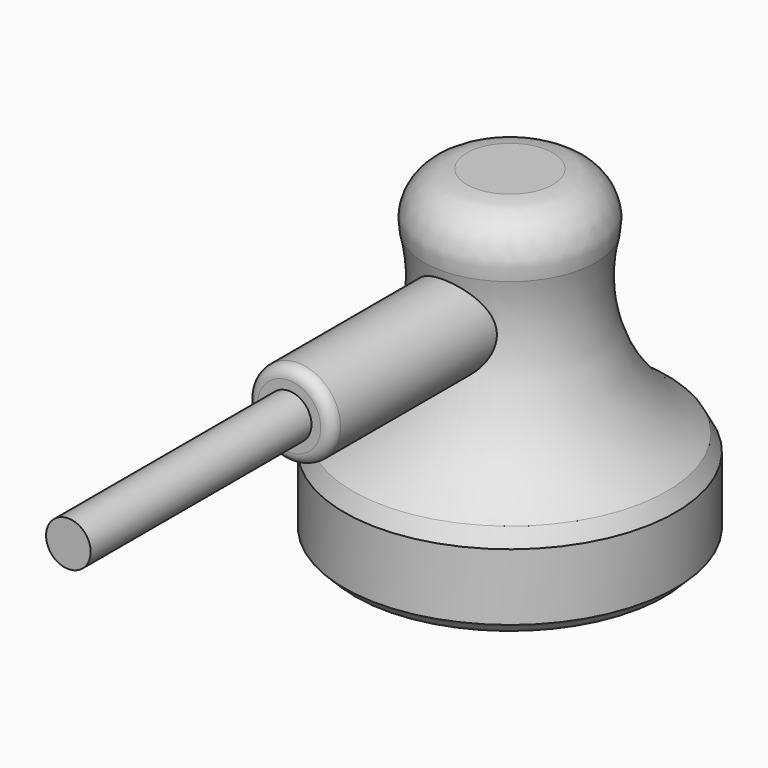
from build123d import *

# Parameters (mm, degrees)
F2_R     = 3.8609958539
F3_DEPTH = 25
F4_R     = 2.0215779579
F5_DEPTH = 25
F6_R     = 4
F8_R     = 1
F9_SIZE  = 1


# Not quite as in the source:
# - a fillet or chamfer that OpenCascade refuses, or shapes differently, is made with other operations: its cross-section is extruded or revolved along the edge and cut away or added


with BuildPart() as f1:
    # F0 (on Front) → F1 (revolve)
    with BuildSketch(Plane.XZ):
        with BuildLine():
            Line((0, 9.6684011082), (0, 39.240504275))
            Line((0, 39.240504275), (-10, 39.240504275))
            ThreePointArc((-10, 39.240504275), (-7.7458675852, 27.3525359295), (-15, 17.6684011082))
            Line((-15, 17.6684011082), (-15, 9.6684011082))
            Line((-15, 9.6684011082), (0, 9.6684011082))
        make_face()
    revolve(axis=Axis((0, 0, 24.4544526916), (0, 0, 1)))

    # F2 (on Front) → F3 (join)
    with BuildSketch(Plane.XZ):
        with Locations((0, 29.6669229865)):
            Circle(F2_R)
    extrude(amount=F3_DEPTH)

    # F4 (on face) → F5 (join)
    with BuildSketch(Plane.XZ.offset(25)):
        with Locations((0, 29.6669229865)):
            Circle(F4_R)
    extrude(amount=F5_DEPTH)

    # F6
    f6_edges = [f1.edges().sort_by_distance(p)[0] for p in [
        (10, 0, 39.240504),
    ]]
    fillet(f6_edges, radius=F6_R)

    # F7: chamfer of 1 on 1 edges, made by hand

    # F7_s1 → F7_t2 (revolve, cut)
    with BuildSketch(Plane.XZ):
        with BuildLine():
            Line((-14.1986684737, 18.1758192127), (-15.0191266727, 16.668849252))
            Line((-15.0191266727, 16.668849252), (-15.0391266727, 16.668849252))
            ThreePointArc((-15.0391266727, 16.668849252), (-15.02, 17.1686251801), (-15.02, 17.6684011082))
            Line((-15.02, 17.6684011082), (-15.00981132, 17.685829189))
            ThreePointArc((-15.00981132, 17.685829189), (-14.6008655323, 17.9246397079), (-14.2095227335, 18.192617577))
            Line((-14.2095227335, 18.192617577), (-14.1986684737, 18.1758192127))
        make_face()
    revolve(axis=Axis((0, 0, 17.6684011082), (0, 0, 1)), mode=Mode.SUBTRACT)

    # F8
    f8_edges = [f1.edges().sort_by_distance(p)[0] for p in [
        (-3.860996, -25, 29.666923),
    ]]
    fillet(f8_edges, radius=F8_R)

    # F9
    f9_edges = [f1.edges().sort_by_distance(p)[0] for p in [
        (15, 0, 9.668401),
    ]]
    chamfer(f9_edges, length=F9_SIZE)


solid = f1.part
